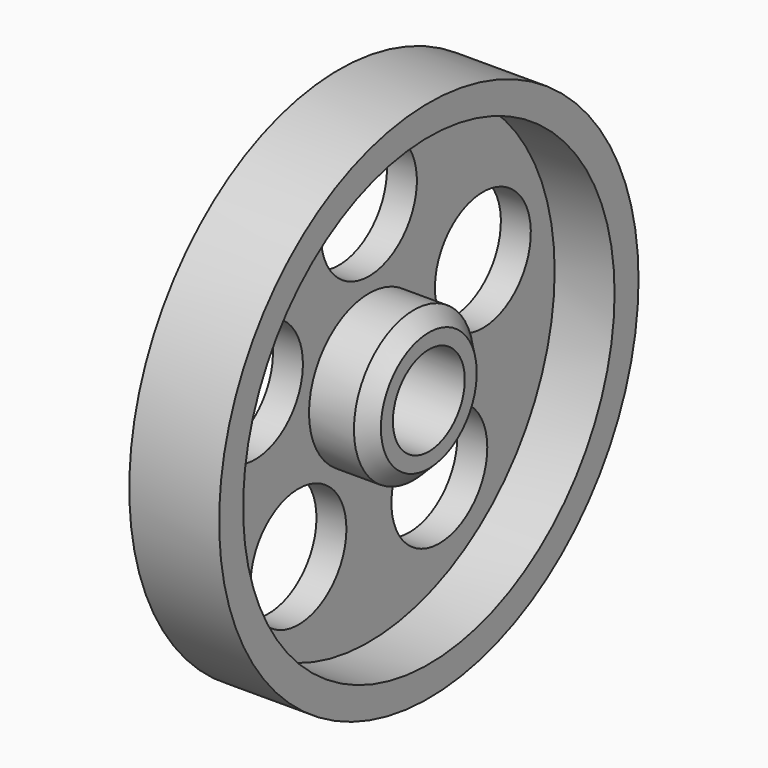
from build123d import *

# Parameters (mm, degrees)
F0_W            = 6
F0_H            = 17.5
F3_D            = 6
F4_T            = -2
F6_D            = 8
F6_COPIES_COUNT = 5
F7_SIZE         = 1


# Not quite as in the source:
# - a pattern or mirror of a feature is missing from the dataset's text; its kind, count and spacing are read off the source's solid


with BuildPart() as f1:
    # F0 (on Top) → F1 (revolve)
    with BuildSketch(Plane.XY):
        with Locations((3, 8.75)):
            Rectangle(F0_W, F0_H)
    revolve(axis=Axis((3, 0, 0), (1, 0, 0)))

    # F3 (through all)
    with Locations(Plane(origin=(0, 0, 0), x_dir=(0, 1, 0), z_dir=(-1, 0, 0))):
        with Locations((0, 0)):
            Hole(F3_D / 2)

    # F4
    f4_openings = [f1.faces().sort_by_distance(p)[0] for p in [
        (6, -17.005025, 0),
    ]]
    offset(amount=F4_T, openings=f4_openings)

    # F6 (through all)
    with Locations(Plane(origin=(0, 0, 0), x_dir=(0, 1, 0), z_dir=(-1, 0, 0))):
        with Locations((0, -10)):
            f6 = Hole(F6_D / 2)

    # F6_copies: F6 ×5 about axis
    f6_copies_axis = Axis((0, 0, 0), (1, 0, 0))
    for i in range(1, F6_COPIES_COUNT):
        add(f6.rotate(f6_copies_axis, i * 360 / F6_COPIES_COUNT), mode=Mode.SUBTRACT)

    # F7
    f7_edges = [f1.edges().sort_by_distance(p)[0] for p in [
        (6, -5, 0),
    ]]
    chamfer(f7_edges, length=F7_SIZE)


solid = f1.part
